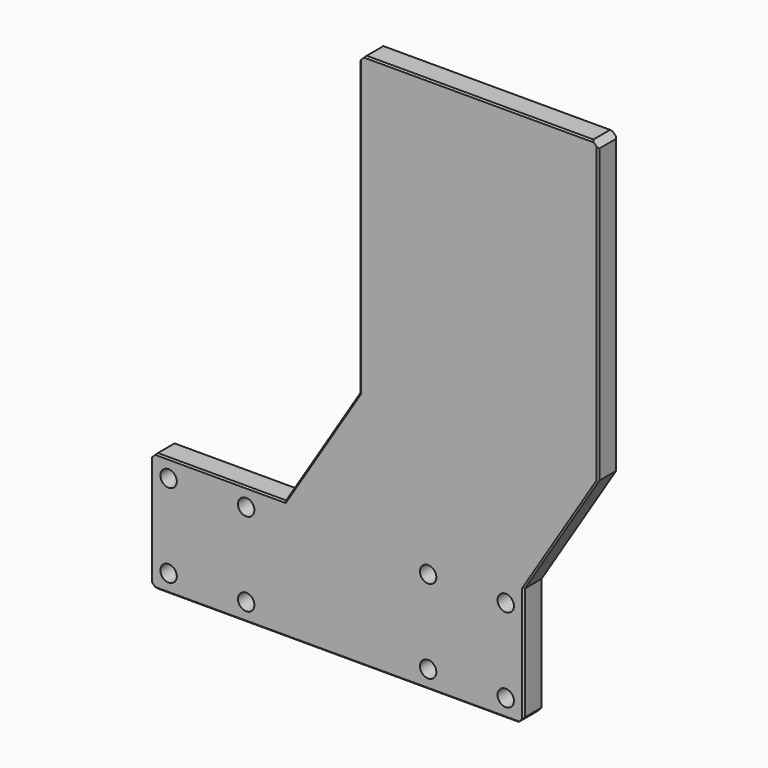
from build123d import *

# Parameters (mm, degrees)
F1_DEPTH    = 8
F3_D        = 5.5
F4_SIZE     = 0.5
F5_T1_DEPTH = 17.2867319519


# Not quite as in the source:
# - a fillet or chamfer that OpenCascade refuses, or shapes differently, is made with other operations: its cross-section is extruded or revolved along the edge and cut away or added


with BuildPart() as f1:
    # F0 (on Front) → F1 (new body)
    with BuildSketch(Plane.XZ):
        Polygon((150, 180), (70, 180), (70, 80), (45, 40), (0, 40), (0, 0), (125, 0), (125, 40), (150, 80), align=None)
    extrude(amount=F1_DEPTH)

    # F3 (through all)
    with Locations(Plane.XZ.offset(8)):
        with Locations((93, 34), (6, 34), (32, 34), (119, 34), (119, 6), (93, 6), (32, 6), (6, 6)):
            Hole(F3_D / 2)

    # F4
    f4_edges = [f1.edges().sort_by_distance(p)[0] for p in [
        (110, -8, 180),
        (70, -8, 130),
        (57.5, -8, 60),
        (22.5, -8, 40),
        (0, -8, 20),
        (62.5, -8, 0),
        (125, -8, 20),
        (137.5, -8, 60),
        (150, -8, 130),
        (110, 0, 180),
        (150, 0, 130),
        (137.5, 0, 60),
        (125, 0, 20),
        (0, 0, 20),
        (22.5, 0, 40),
        (57.5, 0, 60),
        (70, 0, 130),
    ]]
    chamfer(f4_edges, length=F4_SIZE)

    # F5: chamfer of 2 on 5 edges, made by hand

    # F5_s2 → F5_t1 (cut)
    with BuildSketch(Plane.XZ.offset(-4.6433659759)):
        Polygon((72, 180), (70, 178), (70, 180), align=None)
        Polygon((148, 180), (150, 178), (150, 180), align=None)
        Polygon((2, 40), (0, 38), (0, 40), align=None)
        Polygon((2, 0), (0, 2), (0, 0), align=None)
        Polygon((125, 2), (123, 0), (125, 0), align=None)
    extrude(amount=F5_T1_DEPTH, mode=Mode.SUBTRACT)


solid = f1.part
